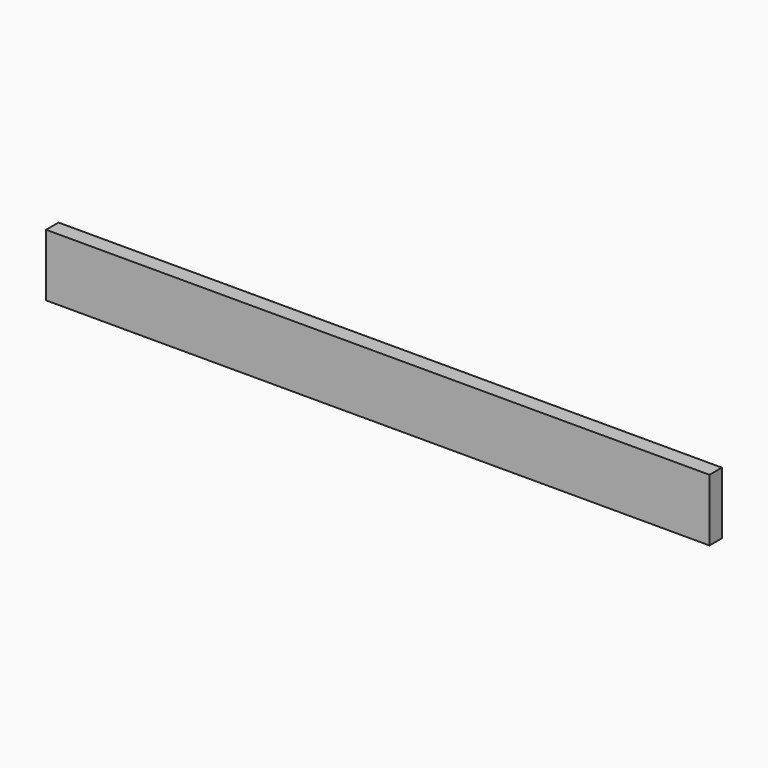
from build123d import *

# Parameters (mm, degrees)
F0_W     = 812.8
F0_H     = 76.2
F1_DEPTH = 19.05


# Not quite as in the source:
# - a feature names something its author has since deleted; it is built from what else it names


with BuildPart() as f1:
    # F0 (on Front) → F1 (new body)
    with BuildSketch(Plane.XZ):
        with Locations((406.4, 38.1)):
            Rectangle(F0_W, F0_H)
    extrude(amount=-F1_DEPTH)


solid = f1.part
